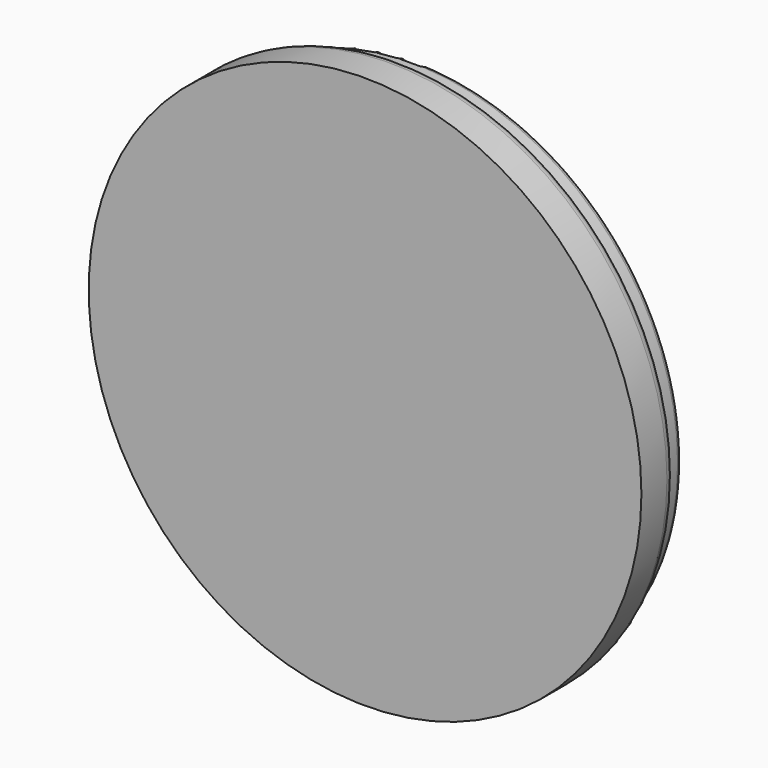
from build123d import *

# Parameters (mm, degrees)
F0_R     = 26
F1_DEPTH = 4
F2_R     = 25
F3_DEPTH = 2
F4_R     = 0.99999
F5_R     = 0.5
F6_W     = 4
F6_H     = 45
F7_DEPTH = 2


# Not quite as in the source:
# - a fillet or chamfer is up to 0.001 mm smaller than in the source, because OpenCascade refuses the exact size


with BuildPart() as f1:
    # F0 (on Front) → F1 (new body)
    with BuildSketch(Plane.XZ):
        Circle(F0_R)
    extrude(amount=F1_DEPTH)

    # F2 (on face) → F3 (join)
    with BuildSketch(Plane(origin=(0, 0, 0), x_dir=(-1, 0, 0), z_dir=(0, 1, 0))):
        Circle(F2_R)
    extrude(amount=F3_DEPTH)

    # F4 (radius 1 in the source; OpenCascade refuses exactly that, so slightly less here)
    f4_edges = [f1.edges().sort_by_distance(p)[0] for p in [
        (-26, 0, 0),
    ]]
    fillet(f4_edges, radius=F4_R)

    # F5
    f5_edges = [f1.edges().sort_by_distance(p)[0] for p in [
        (25, 2, 0),
    ]]
    fillet(f5_edges, radius=F5_R)

    # F6 (on face) → F7 (cut)
    with BuildSketch(Plane(origin=(0, 2, 0), x_dir=(-1, 0, 0), z_dir=(0, 1, 0))):
        Rectangle(F6_W, F6_H)
    extrude(amount=-F7_DEPTH, mode=Mode.SUBTRACT)


solid = f1.part
